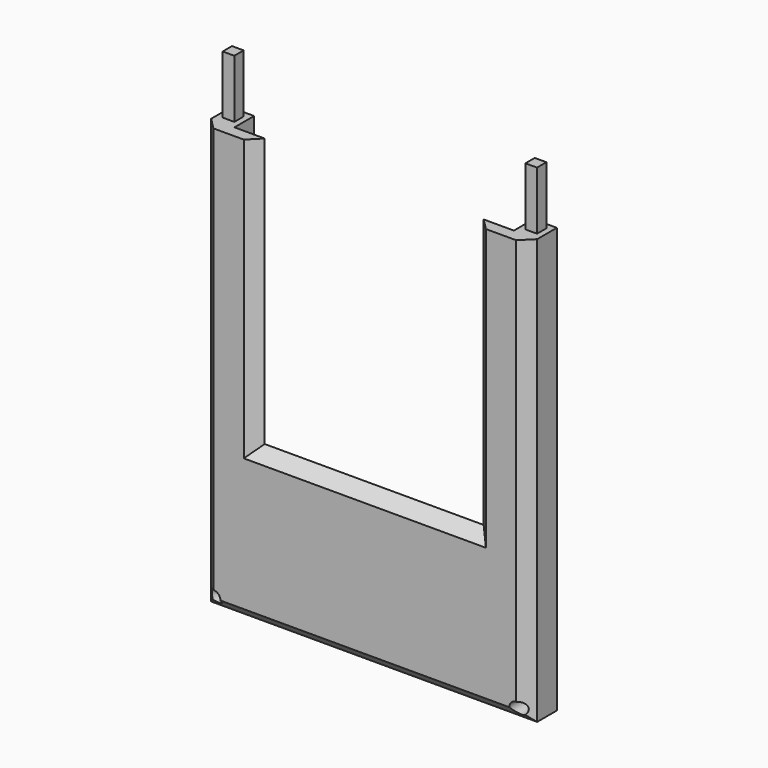
from build123d import *

# Parameters (mm, degrees)
F0_W        = 140
F0_H        = 252.5
F0_R        = 1
F0_W_2      = 94
F0_H_2      = 152.5
F0_R_2      = 2.5
F0_W_3      = 12
F0_H_3      = 34
F1_DEPTH    = 15.56
F2_DEPTH    = 10.56
F3_T1_DEPTH = 165.7168298797
F3_T3_DEPTH = 278.2168298797
F4_SIZE     = 2.5
F5_R        = 3
F6_DEPTH    = 10
F7_SIZE     = 4.99999
F8_W        = 161.2529857084
F8_H        = 70
F9_DEPTH    = 25
F11_W       = 5
F11_H       = 50
F12_DEPTH   = 5


# Not quite as in the source:
# - a fillet or chamfer that OpenCascade refuses, or shapes differently, is made with other operations: its cross-section is extruded or revolved along the edge and cut away or added
# - a fillet or chamfer is up to 0.001 mm smaller than in the source, because OpenCascade refuses the exact size
# - a feature names something its author has since deleted; it is built from what else it names


with BuildPart() as f1:
    # F0 (on Front) → F1 (new body)
    with BuildSketch(Plane.XZ):
        with Locations((-70, 126.25)):
            Rectangle(F0_W, F0_H)
        with Locations((-135, 5)):
            Circle(F0_R, mode=Mode.SUBTRACT)
        with Locations((-5, 5)):
            Circle(F0_R, mode=Mode.SUBTRACT)
        with Locations((-135, 247.5)):
            Circle(F0_R, mode=Mode.SUBTRACT)
        Polygon((-130, 44), (-130, 242.5), (-10, 242.5), (-10, 44), (-64, 44), (-64, 10), (-76, 10), (-76, 44), align=None, mode=Mode.SUBTRACT)
        with Locations((-5, 247.5)):
            Circle(F0_R, mode=Mode.SUBTRACT)
        Polygon((-10, 242.5), (-130, 242.5), (-130, 44), (-76, 44), (-64, 44), (-10, 44), align=None)
        with Locations((-70, 143.25)):
            Rectangle(F0_W_2, F0_H_2, mode=Mode.SUBTRACT)
        with Locations((-70, 232.5)):
            Circle(F0_R_2, mode=Mode.SUBTRACT)
        with Locations((-70, 27)):
            Rectangle(F0_W_3, F0_H_3)
    extrude(amount=F1_DEPTH)

    # F0 (on Front) → F2 (cut)
    with BuildSketch(Plane.XZ):
        Polygon((-10, 242.5), (-130, 242.5), (-130, 44), (-76, 44), (-64, 44), (-10, 44), align=None)
        with Locations((-70, 143.25)):
            Rectangle(F0_W_2, F0_H_2, mode=Mode.SUBTRACT)
        with Locations((-70, 232.5)):
            Circle(F0_R_2, mode=Mode.SUBTRACT)
        with Locations((-70, 27)):
            Rectangle(F0_W_3, F0_H_3)
    extrude(amount=F2_DEPTH, mode=Mode.SUBTRACT)

    # F3: chamfer of 5 on 4 edges, made by hand

    # F3_s2 → F3_t1 (cut)
    with BuildSketch(Plane.YZ.offset(-152.8584149398)):
        Polygon((-10.56, 0), (-15.56, 5), (-15.56, 0), align=None)
        Polygon((-15.56, 247.5), (-10.56, 252.5), (-15.56, 252.5), align=None)
    extrude(amount=F3_T1_DEPTH, mode=Mode.SUBTRACT)

    # F3_s4 → F3_t3 (cut)
    with BuildSketch(Plane.XY.offset(-12.8584149398)):
        Polygon((-140, -10.56), (-135, -15.56), (-140, -15.56), align=None)
        Polygon((0, -10.56), (-5, -15.56), (0, -15.56), align=None)
    extrude(amount=F3_T3_DEPTH, mode=Mode.SUBTRACT)

    # F4
    f4_edges = [f1.edges().sort_by_distance(p)[0] for p in [
        (-72.5, -15.56, 232.5),
    ]]
    chamfer(f4_edges, length=F4_SIZE)

    # F5 (on face) → F6 (cut)
    with BuildSketch(Plane.XZ.offset(15.56)):
        with Locations((-135, 247.5)):
            Circle(F5_R)
        with Locations((-135, 5)):
            Circle(F5_R)
        with Locations((-5, 247.5)):
            Circle(F5_R)
        with Locations((-5, 5)):
            Circle(F5_R)
    extrude(amount=-F6_DEPTH, mode=Mode.SUBTRACT)

    # F7 (size 5 in the source; OpenCascade refuses exactly that, so slightly less here)
    f7_edges = [f1.edges().sort_by_distance(p)[0] for p in [
        (-70, -15.56, 67),
        (-117, -15.56, 143.25),
        (-23, -15.56, 143.25),
        (-70, -15.56, 219.5),
    ]]
    chamfer(f7_edges, length=F7_SIZE)

    # F8 (on face) → F9 (cut)
    with BuildSketch(Plane.XZ.offset(15.56)):
        with Locations((-74.815297965, 217.5)):
            Rectangle(F8_W, F8_H)
    extrude(amount=-F9_DEPTH, mode=Mode.SUBTRACT)

    # F11 (on offset) → F12 (join)
    with BuildSketch(Plane(origin=(0, -2.5, 0), x_dir=(-1, 0, 0), z_dir=(0, 1, 0))):
        with Locations((135, 182.5)):
            Rectangle(F11_W, F11_H)
        with Locations((5, 182.5)):
            Rectangle(F11_W, F11_H)
    extrude(amount=-F12_DEPTH)


solid = f1.part
